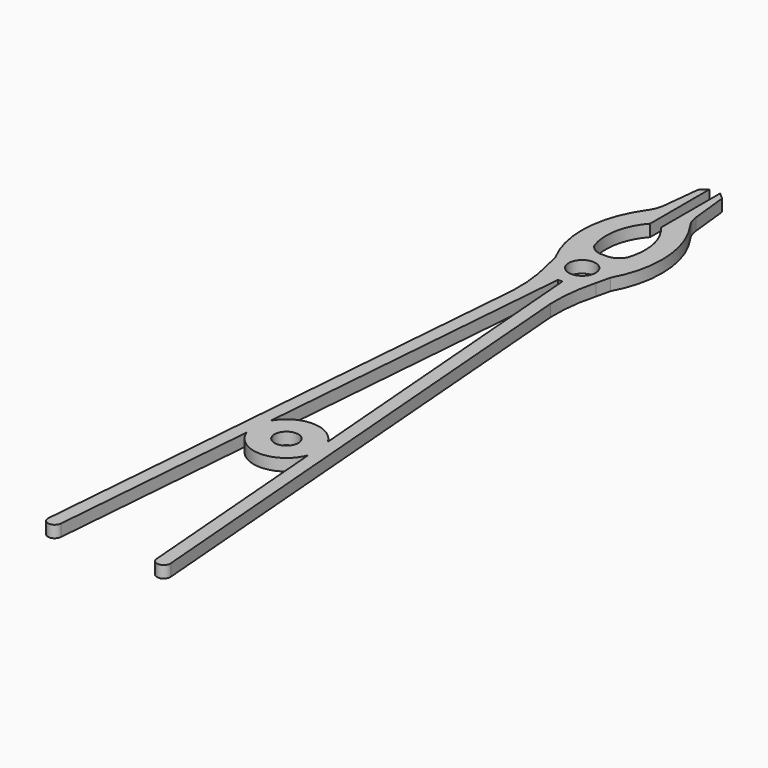
from build123d import *

# Parameters (mm, degrees)
F0_R     = 2
F0_R_2   = 2.2544770367
F1_DEPTH = 2


# Not quite as in the source:
# - ends of sketch curves that miss each other by under 0.0002 mm in the source are joined


with BuildPart() as f1:
    # F0 (on Top) → F1 (new body)
    with BuildSketch(Plane.XY):
        with BuildLine():
            ThreePointArc((-5.1683257468, -1.8810659147), (0, -5.5), (5.1683257468, -1.8810659147))
            Line((5.1683257468, -1.8810659147), (8.0301481547, -37.2918741238))
            ThreePointArc((8.0301481547, -37.2918741238), (9.2788304803, -38.3188106152), (10.2640215975, -37.0369352038))
            Line((10.2640215975, -37.0369352038), (3.1098692343, 51.4850906656))
            ThreePointArc((3.1098692343, 51.4850906656), (3.2758505583, 55.7142948477), (4.0791085727, 59.8698326439))
            Line((4.0791085727, 59.8698326439), (4.6310273864, 62.2435739623))
            ThreePointArc((4.6310273864, 62.2435739623), (6.6977396132, 71.4003991777), (3.5793046773, 80.2544440729))
            ThreePointArc((3.5793046773, 80.2544440729), (2.9779070013, 81.3790562482), (2.6805769718, 82.6192282376))
            Line((2.6805769718, 82.6192282376), (2.0130627379, 88.8089160456))
            ThreePointArc((2.0130627379, 88.8089160456), (1.9844093078, 88.9043745509), (1.9233044553, 88.9831117232))
            Line((1.9233044553, 88.9831117232), (0.9, 89.8927152157))
            Line((0.9, 89.8927152157), (0.9, 77.4665676321))
            ThreePointArc((0.9, 77.4665676321), (3.1034376701, 73.0014155649), (2.7328648238, 68.0359955106))
            ThreePointArc((2.7328648238, 68.0359955106), (1.8069828059, 67.0668885057), (0.5256445201, 66.6736988627))
            ThreePointArc((0.5256445201, 66.6736988627), (0.2620789214, 66.6755874914), (0, 66.7036058899))
            ThreePointArc((0, 66.7036058899), (-0.2620789214, 66.6755874914), (-0.5256445201, 66.6736988627))
            ThreePointArc((-0.5256445201, 66.6736988627), (-1.8069828059, 67.0668885057), (-2.7328648238, 68.0359955106))
            ThreePointArc((-2.7328648238, 68.0359955106), (-3.1034376701, 73.0014155649), (-0.9, 77.4665676321))
            Line((-0.9, 77.4665676321), (-0.9, 89.8927152157))
            Line((-0.9, 89.8927152157), (-1.9233044553, 88.9831117232))
            ThreePointArc((-1.9233044553, 88.9831117232), (-1.9844093078, 88.9043745509), (-2.0130627379, 88.8089160456))
            Line((-2.0130627379, 88.8089160456), (-2.6805769718, 82.6192282376))
            ThreePointArc((-2.6805769718, 82.6192282376), (-2.9779070013, 81.3790562482), (-3.5793046773, 80.2544440729))
            ThreePointArc((-3.5793046773, 80.2544440729), (-6.6977396132, 71.4003991777), (-4.6310273864, 62.2435739623))
            Line((-4.6310273864, 62.2435739623), (-4.0791085727, 59.8698326439))
            ThreePointArc((-4.0791085727, 59.8698326439), (-3.2758505583, 55.7142948477), (-3.1098692343, 51.4850906656))
            Line((-3.1098692343, 51.4850906656), (-10.2640215975, -37.0369352038))
            Line((-10.2640215975, -37.0369352038), (-10.264126962, -37.0382389339))
            ThreePointArc((-10.264126962, -37.0382389339), (-9.2781820506, -38.3188844261), (-8.0301481547, -37.2918741238))
            Line((-8.0301481547, -37.2918741238), (-5.1683257468, -1.8810659147))
        make_face()
        Circle(F0_R, mode=Mode.SUBTRACT)
        with BuildLine():
            ThreePointArc((4.7991758084, 2.6866171219), (0, 5.5), (-4.7991758084, 2.6866171219))
            Line((-4.7991758084, 2.6866171219), (-0.3733170252, 57.4500560059))
            ThreePointArc((-0.3733170252, 57.4500560059), (0, 57.4349952343), (0.3733170252, 57.4500560059))
            Line((0.3733170252, 57.4500560059), (4.7991758084, 2.6866171219))
        make_face(mode=Mode.SUBTRACT)
        with Locations((0, 62.0693005621)):
            Circle(F0_R_2, mode=Mode.SUBTRACT)
    extrude(amount=F1_DEPTH)


solid = f1.part
